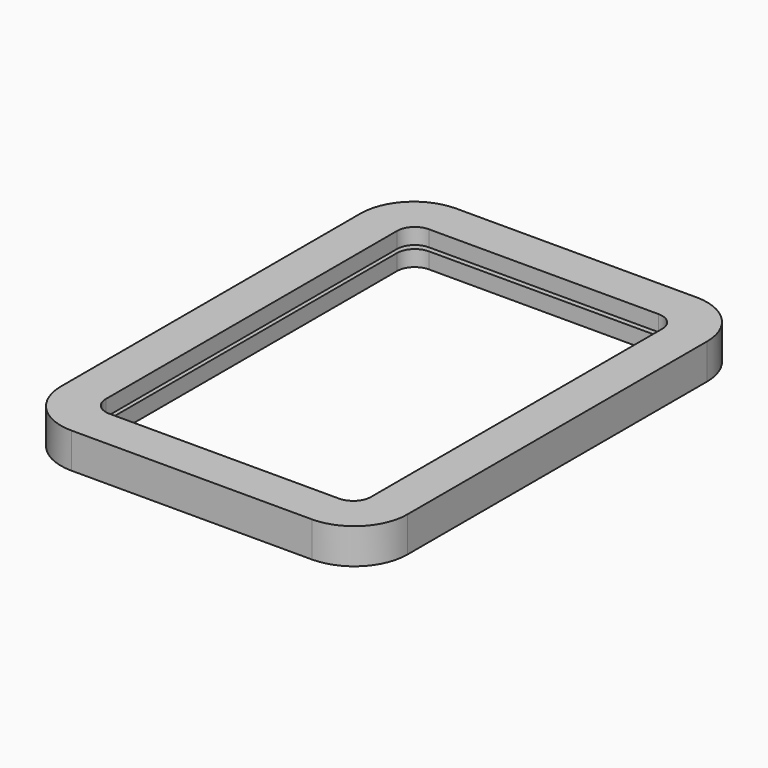
from build123d import *

# Parameters (mm, degrees)
F0_W        = 98
F0_H        = 136
F0_W_2      = 78
F0_H_2      = 116
F0_W_3      = 75
F0_H_3      = 113
F1_DEPTH    = 5
F2_W        = 78
F2_H        = 130
F3_DEPTH    = 0.5
F5_T1_DEPTH = 85
F6_R        = 5


# Not quite as in the source:
# - a fillet or chamfer that OpenCascade refuses, or shapes differently, is made with other operations: its cross-section is extruded or revolved along the edge and cut away or added
# - a feature of the source that left no trace in its solid (it failed there, or was rolled back) is left out


with BuildPart() as f1:
    # F0 (on Top) → F1 (new body, symmetric)
    with BuildSketch(Plane.XY):
        Rectangle(F0_W, F0_H)
        Rectangle(F0_W_2, F0_H_2, mode=Mode.SUBTRACT)
        Rectangle(F0_W_2, F0_H_2)
        Rectangle(F0_W_3, F0_H_3, mode=Mode.SUBTRACT)
    extrude(amount=F1_DEPTH, both=True)

    # F2 (on Top) → F3 (cut, symmetric)
    with BuildSketch(Plane.XY):
        with Locations((0, 7)):
            Rectangle(F2_W, F2_H)
    extrude(amount=F3_DEPTH, both=True, mode=Mode.SUBTRACT)

    # F5: fillet of radius 15 on 4 edges, made by hand

    # F5_s2 → F5_t1 (cut)
    with BuildSketch(Plane.XY.offset(-42.5)):
        with BuildLine():
            ThreePointArc((-34, -68), (-44.6066017178, -63.6066017178), (-49, -53))
            Line((-49, -53), (-49, -68))
            Line((-49, -68), (-34, -68))
        make_face()
        with BuildLine():
            ThreePointArc((34, -68), (44.6066017178, -63.6066017178), (49, -53))
            Line((49, -53), (49, -68))
            Line((49, -68), (34, -68))
        make_face()
        with BuildLine():
            ThreePointArc((34, 68), (44.6066017178, 63.6066017178), (49, 53))
            Line((49, 53), (49, 68))
            Line((49, 68), (34, 68))
        make_face()
        with BuildLine():
            ThreePointArc((-34, 68), (-44.6066017178, 63.6066017178), (-49, 53))
            Line((-49, 53), (-49, 68))
            Line((-49, 68), (-34, 68))
        make_face()
    extrude(amount=F5_T1_DEPTH, mode=Mode.SUBTRACT)

    # F6
    f6_edges = [f1.edges().sort_by_distance(p)[0] for p in [
        (37.5, -56.5, -2.75),
        (37.5, -56.5, 2.75),
        (-37.5, -56.5, 2.75),
        (-37.5, -56.5, -2.75),
        (-37.5, 56.5, 2.75),
        (-37.5, 56.5, -2.75),
        (37.5, 56.5, -2.75),
        (37.5, 56.5, 2.75),
    ]]
    fillet(f6_edges, radius=F6_R)


solid = f1.part
